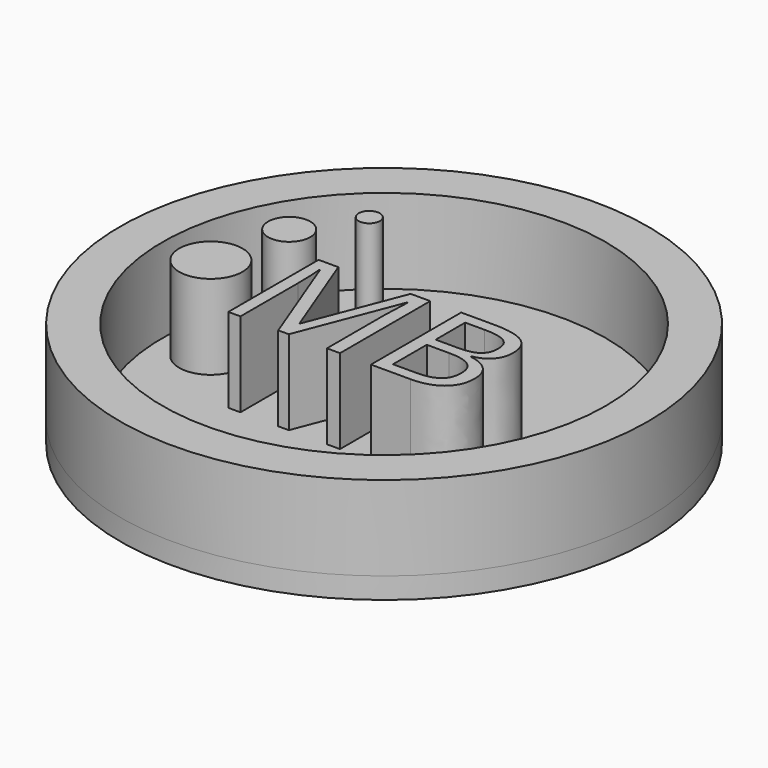
from build123d import *

# Parameters (mm, degrees)
F0_R         = 25
F0_R_2       = 21
F0_TEXT_SIZE = 14.9608686722
F0_R_3       = 2
F0_R_4       = 1
F0_R_5       = 3
F1_DEPTH     = 8
F2_R         = 25
F3_DEPTH     = 2


# Not quite as in the source:
# - Text() gives the source's letters only with a copy of the font that has no kerning and outlines rounded to 1/6400 em; it was checked with that copy


with BuildPart() as f1:
    # F0 (on Top) → F1 (new body)
    with BuildSketch(Plane.XY):
        Circle(F0_R)
        Circle(F0_R_2, mode=Mode.SUBTRACT)
        with Locations((-11.6729840179, -5.6826160289)):
            Text('MB', F0_TEXT_SIZE, font='Open Sans', text_align=(TextAlign.LEFT, TextAlign.BOTTOM))
        with Locations((-14.9501100803, 7.4555913443)):
            Circle(F0_R_3)
        with Locations((-11.5482881665, 12.6808062196)):
            Circle(F0_R_4)
        with Locations((-16.3933963316, -0.0200778211)):
            Circle(F0_R_5)
    extrude(amount=F1_DEPTH)


with BuildPart() as f3:
    # F2 (on Top) → F3 (new body)
    with BuildSketch(Plane.XY):
        Circle(F2_R)
    extrude(amount=-F3_DEPTH)


solid = Compound([f1.part, f3.part])
